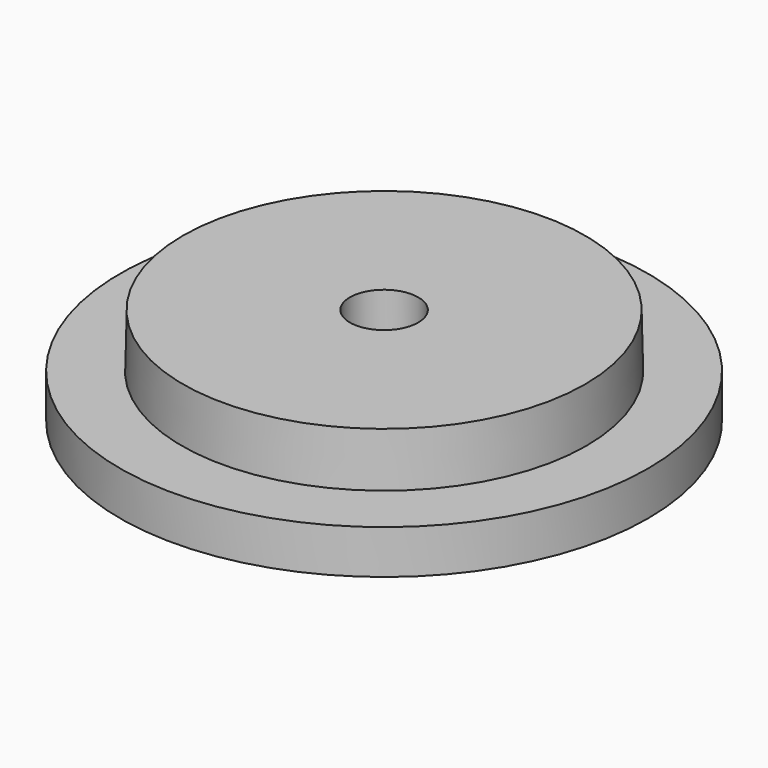
from build123d import *

# Parameters (mm, degrees)
F0_R     = 61.3
F1_DEPTH = 10.2
F2_R     = 47
F3_DEPTH = 12.5
F4_SIZE2 = 12.49999
F4_SIZE  = 0.27999
F5_R     = 7.9375
F6_DEPTH = 22.701


# Not quite as in the source:
# - a fillet or chamfer is up to 0.001 mm smaller than in the source, because OpenCascade refuses the exact size


with BuildPart() as f1:
    # F0 (on Top) → F1 (new body)
    with BuildSketch(Plane.XY):
        Circle(F0_R)
    extrude(amount=F1_DEPTH)

    # F2 (on face) → F3 (join)
    with BuildSketch(Plane.XY.offset(10.2)):
        Circle(F2_R)
    extrude(amount=F3_DEPTH)

    # F4 (size 0.28 and 12.5 in the source; OpenCascade refuses exactly that, so slightly less here)
    f4_edges = [f1.edges().sort_by_distance(p)[0] for p in [
        (-47, 0, 22.7),
    ]]
    f4_side = f1.faces().sort_by_distance((0, 0, 22.7))[0]
    chamfer(f4_edges, length=F4_SIZE, length2=F4_SIZE2, reference=f4_side)

    # F5 (on face) → F6 (cut, through all)
    with BuildSketch(Plane.XY.offset(22.7)):
        Circle(F5_R)
    extrude(amount=-F6_DEPTH, mode=Mode.SUBTRACT)


solid = f1.part
